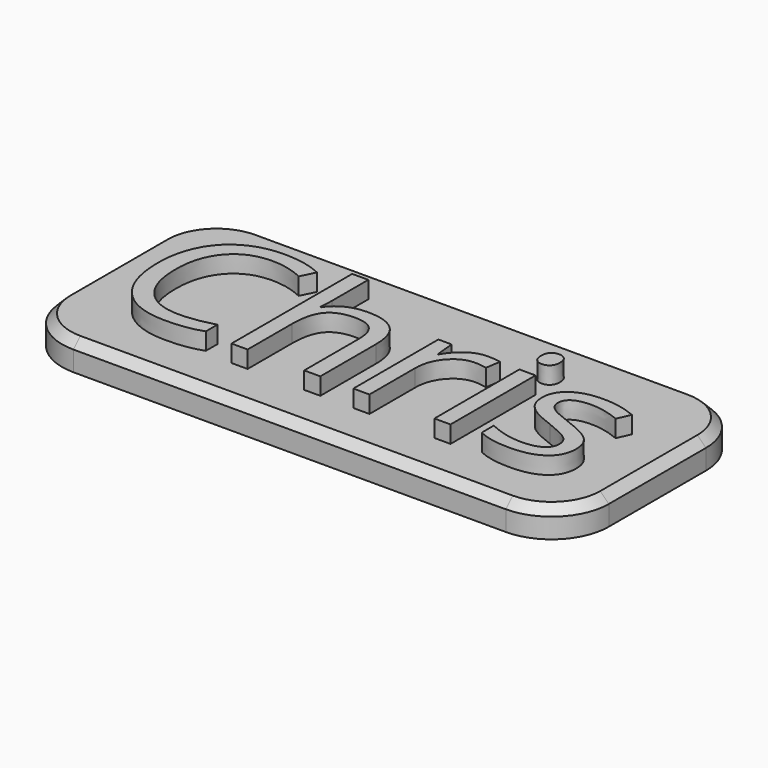
from build123d import *

# Parameters (mm, degrees)
F0_W         = 95.6249979794
F0_H         = 41.2499999501
F0_W_2       = 2.8157552083
F0_H_2       = 18.5818142361
F0_TEXT_SIZE = 34.7222222222
F1_DEPTH     = 5
F2_DEPTH     = 8
F3_R         = 10
F4_SIZE      = 1.5


# Not quite as in the source:
# - Text() gives the source's letters only with a copy of the font that has no kerning and outlines rounded to 1/6400 em; it was checked with that copy


with BuildPart() as f1:
    # F0 (on Top) → F1 (new body)
    with BuildSketch(Plane.XY):
        with Locations((6.9999974221, -3.5000005737)):
            Rectangle(F0_W, F0_H)
        with BuildLine():
            add(Edge.make_bspline(
                [(-14.9118961738, 5.2456596475), (-17.7276513822, 6.5640190225), (-20.5434065905, 6.5640190225)],
                knots=[0, 0, 0, 1, 1, 1], degree=2))
            add(Edge.make_bspline(
                [(-20.5434065905, 6.5640190225), (-24.6286930488, 6.5640190225), (-26.9941444377, 3.8432073905)],
                knots=[0, 0, 0, 1, 1, 1], degree=2))
            add(Edge.make_bspline(
                [(-26.9941444377, 3.8432073905), (-29.3595958266, 1.1223957586), (-29.3595958266, -3.6085070192)],
                knots=[0, 0, 0, 1, 1, 1], degree=2))
            add(Edge.make_bspline(
                [(-29.3595958266, -3.6085070192), (-29.3595958266, -8.4696181303), (-27.0782373197, -11.1253255956)],
                knots=[0, 0, 0, 1, 1, 1], degree=2))
            add(Edge.make_bspline(
                [(-27.0782373197, -11.1253255956), (-24.7968788127, -13.7810330609), (-20.5759586738, -13.7810330609)],
                knots=[0, 0, 0, 1, 1, 1], degree=2))
            add(Edge.make_bspline(
                [(-20.5759586738, -13.7810330609), (-17.9826427016, -13.7810330609), (-14.6569048544, -12.8478733387)],
                knots=[0, 0, 0, 1, 1, 1], degree=2))
            Line((-14.6569048544, -12.8478733387), (-14.6569048544, -15.370659797))
            add(Edge.make_bspline(
                [(-14.6569048544, -15.370659797), (-17.233944785, -16.3417969498), (-21.0154117988, -16.3417969498)],
                knots=[0, 0, 0, 1, 1, 1], degree=2))
            add(Edge.make_bspline(
                [(-21.0154117988, -16.3417969498), (-26.4895871461, -16.3417969498), (-29.4653900975, -13.0160591025)],
                knots=[0, 0, 0, 1, 1, 1], degree=2))
            add(Edge.make_bspline(
                [(-29.4653900975, -13.0160591025), (-32.4411930488, -9.6903212553), (-32.4411930488, -3.5705295887)],
                knots=[0, 0, 0, 1, 1, 1], degree=2))
            add(Edge.make_bspline(
                [(-32.4411930488, -3.5705295887), (-32.4411930488, 0.2597655502), (-31.0089013822, 3.1406249252)],
                knots=[0, 0, 0, 1, 1, 1], degree=2))
            add(Edge.make_bspline(
                [(-31.0089013822, 3.1406249252), (-29.5766097155, 6.0214843002), (-26.8720741252, 7.5812716266)],
                knots=[0, 0, 0, 1, 1, 1], degree=2))
            add(Edge.make_bspline(
                [(-26.8720741252, 7.5812716266), (-24.167538535, 9.141058953), (-20.50542916, 9.141058953)],
                knots=[0, 0, 0, 1, 1, 1], degree=2))
            add(Edge.make_bspline(
                [(-20.50542916, 9.141058953), (-16.6100298544, 9.141058953), (-13.6911930488, 7.7196179808)],
                knots=[0, 0, 0, 1, 1, 1], degree=2))
            Line((-13.6911930488, 7.7196179808), (-14.9118961738, 5.2456596475))
        make_face(mode=Mode.SUBTRACT)
        with BuildLine():
            add(Edge.make_bspline(
                [(16.9131906317, 1.9389105155), (18.3726090345, 2.9236110363), (20.11957084, 2.9236110363)],
                knots=[0, 0, 0, 1, 1, 1], degree=2))
            add(Edge.make_bspline(
                [(20.11957084, 2.9236110363), (21.3565500067, 2.9236110363), (22.3385378539, 2.7174478419)],
                knots=[0, 0, 0, 1, 1, 1], degree=2))
            Line((22.3385378539, 2.7174478419), (21.9479128539, 0.107855828))
            add(Edge.make_bspline(
                [(21.9479128539, 0.107855828), (20.7977392428, 0.3628471475), (19.9134076456, 0.3628471475)],
                knots=[0, 0, 0, 1, 1, 1], degree=2))
            add(Edge.make_bspline(
                [(19.9134076456, 0.3628471475), (17.6564632012, 0.3628471475), (16.0559857706, -1.46820754)],
                knots=[0, 0, 0, 1, 1, 1], degree=2))
            add(Edge.make_bspline(
                [(16.0559857706, -1.46820754), (14.45550834, -3.2992622275), (14.45550834, -6.0282118803)],
                knots=[0, 0, 0, 1, 1, 1], degree=2))
            Line((14.45550834, -6.0282118803), (14.45550834, -16.0000000748))
            Line((14.45550834, -16.0000000748), (11.6397531317, -16.0000000748))
            Line((11.6397531317, -16.0000000748), (11.6397531317, 2.5818141613))
            Line((11.6397531317, 2.5818141613), (13.9618017428, 2.5818141613))
            Line((13.9618017428, 2.5818141613), (14.2873225762, -0.8578559775))
            Line((14.2873225762, -0.8578559775), (14.4229562567, -0.8578559775))
            add(Edge.make_bspline(
                [(14.4229562567, -0.8578559775), (15.4537722289, 0.9542099947), (16.9131906317, 1.9389105155)],
                knots=[0, 0, 0, 1, 1, 1], degree=2))
        make_face(mode=Mode.SUBTRACT)
        with Locations((27.2240630275, -6.7090929567)):
            Rectangle(F0_W_2, F0_H_2, mode=Mode.SUBTRACT)
        with BuildLine():
            add(Edge.make_bspline(
                [(45.4233902845, -7.8619792414), (46.58441459, -9.0826823664), (46.58441459, -10.9327257692)],
                knots=[0, 0, 0, 1, 1, 1], degree=2))
            add(Edge.make_bspline(
                [(46.58441459, -10.9327257692), (46.58441459, -13.5260417414), (44.6529909789, -14.9339193456)],
                knots=[0, 0, 0, 1, 1, 1], degree=2))
            add(Edge.make_bspline(
                [(44.6529909789, -14.9339193456), (42.7215673678, -16.3417969498), (39.2276437567, -16.3417969498)],
                knots=[0, 0, 0, 1, 1, 1], degree=2))
            add(Edge.make_bspline(
                [(39.2276437567, -16.3417969498), (35.5329822984, -16.3417969498), (33.4659250067, -15.1699219498)],
                knots=[0, 0, 0, 1, 1, 1], degree=2))
            Line((33.4659250067, -15.1699219498), (33.4659250067, -12.5603299359))
            add(Edge.make_bspline(
                [(33.4659250067, -12.5603299359), (34.8059857706, -13.2384983387), (36.3386463609, -13.626410665)],
                knots=[0, 0, 0, 1, 1, 1], degree=2))
            add(Edge.make_bspline(
                [(36.3386463609, -13.626410665), (37.8713069512, -14.0143229914), (39.2981732706, -14.0143229914)],
                knots=[0, 0, 0, 1, 1, 1], degree=2))
            add(Edge.make_bspline(
                [(39.2981732706, -14.0143229914), (41.5008642428, -14.0143229914), (42.6863026109, -13.3117405262)],
                knots=[0, 0, 0, 1, 1, 1], degree=2))
            add(Edge.make_bspline(
                [(42.6863026109, -13.3117405262), (43.8717409789, -12.6091580609), (43.8717409789, -11.1660156998)],
                knots=[0, 0, 0, 1, 1, 1], degree=2))
            add(Edge.make_bspline(
                [(43.8717409789, -11.1660156998), (43.8717409789, -10.0809462553), (42.9331559095, -9.3105469498)],
                knots=[0, 0, 0, 1, 1, 1], degree=2))
            add(Edge.make_bspline(
                [(42.9331559095, -9.3105469498), (41.99457084, -8.5401476442), (39.26019584, -7.4876302831)],
                knots=[0, 0, 0, 1, 1, 1], degree=2))
            add(Edge.make_bspline(
                [(39.26019584, -7.4876302831), (36.6668798678, -6.5219184775), (35.5736724025, -5.800347297)],
                knots=[0, 0, 0, 1, 1, 1], degree=2))
            add(Edge.make_bspline(
                [(35.5736724025, -5.800347297), (34.4804649373, -5.0787761164), (33.9460682359, -4.1646051095)],
                knots=[0, 0, 0, 1, 1, 1], degree=2))
            add(Edge.make_bspline(
                [(33.9460682359, -4.1646051095), (33.4116715345, -3.2504341025), (33.4116715345, -1.9809028525)],
                knots=[0, 0, 0, 1, 1, 1], degree=2))
            add(Edge.make_bspline(
                [(33.4116715345, -1.9809028525), (33.4116715345, 0.2923176336), (35.2617149373, 1.607964335)],
                knots=[0, 0, 0, 1, 1, 1], degree=2))
            add(Edge.make_bspline(
                [(35.2617149373, 1.607964335), (37.11175834, 2.9236110363), (40.3289892428, 2.9236110363)],
                knots=[0, 0, 0, 1, 1, 1], degree=2))
            add(Edge.make_bspline(
                [(40.3289892428, 2.9236110363), (43.3292062567, 2.9236110363), (46.1992149373, 1.7029079113)],
                knots=[0, 0, 0, 1, 1, 1], degree=2))
            Line((46.1992149373, 1.7029079113), (45.1955257012, -0.5865886164))
            add(Edge.make_bspline(
                [(45.1955257012, -0.5865886164), (42.4014718817, 0.5635849947), (40.1282513956, 0.5635849947)],
                knots=[0, 0, 0, 1, 1, 1], degree=2))
            add(Edge.make_bspline(
                [(40.1282513956, 0.5635849947), (38.1262982706, 0.5635849947), (37.1090456664, -0.0630426095)],
                knots=[0, 0, 0, 1, 1, 1], degree=2))
            add(Edge.make_bspline(
                [(37.1090456664, -0.0630426095), (36.0917930623, -0.6896702137), (36.0917930623, -1.7910156998)],
                knots=[0, 0, 0, 1, 1, 1], degree=2))
            add(Edge.make_bspline(
                [(36.0917930623, -1.7910156998), (36.0917930623, -2.5397136164), (36.4742800414, -3.0632596234)],
                knots=[0, 0, 0, 1, 1, 1], degree=2))
            add(Edge.make_bspline(
                [(36.4742800414, -3.0632596234), (36.8567670206, -3.5868056303), (37.7031211873, -4.0615235123)],
                knots=[0, 0, 0, 1, 1, 1], degree=2))
            add(Edge.make_bspline(
                [(37.7031211873, -4.0615235123), (38.5494753539, -4.5362413942), (40.9583295206, -5.4368490331)],
                knots=[0, 0, 0, 1, 1, 1], degree=2))
            add(Edge.make_bspline(
                [(40.9583295206, -5.4368490331), (44.2623659789, -6.6412761164), (45.4233902845, -7.8619792414)],
                knots=[0, 0, 0, 1, 1, 1], degree=2))
        make_face(mode=Mode.SUBTRACT)
        with BuildLine():
            Line((5.86175834, -16.0000000748), (3.0460031317, -16.0000000748))
            Line((3.0460031317, -16.0000000748), (3.0460031317, -3.9774306303))
            add(Edge.make_bspline(
                [(3.0460031317, -3.9774306303), (3.0460031317, -1.7096354914), (2.0124744859, -0.58930129)],
                knots=[0, 0, 0, 1, 1, 1], degree=2))
            add(Edge.make_bspline(
                [(2.0124744859, -0.58930129), (0.97894584, 0.5310329113), (-1.2291704794, 0.5310329113)],
                knots=[0, 0, 0, 1, 1, 1], degree=2))
            add(Edge.make_bspline(
                [(-1.2291704794, 0.5310329113), (-4.1588579794, 0.5310329113), (-5.5070567641, -1.064019172)],
                knots=[0, 0, 0, 1, 1, 1], degree=2))
            add(Edge.make_bspline(
                [(-5.5070567641, -1.064019172), (-6.8552555488, -2.6590712553), (-6.8552555488, -6.2832031998)],
                knots=[0, 0, 0, 1, 1, 1], degree=2))
            Line((-6.8552555488, -6.2832031998), (-6.8552555488, -16.0000000748))
            Line((-6.8552555488, -16.0000000748), (-9.6710107572, -16.0000000748))
            Line((-9.6710107572, -16.0000000748), (-9.6710107572, 10.3834634669))
            Line((-9.6710107572, 10.3834634669), (-6.8552555488, 10.3834634669))
            Line((-6.8552555488, 10.3834634669), (-6.8552555488, 2.3973523558))
            add(Edge.make_bspline(
                [(-6.8552555488, 2.3973523558), (-6.8552555488, 0.9542099947), (-6.9908892294, 0.0047742308)],
                knots=[0, 0, 0, 1, 1, 1], degree=2))
            Line((-6.9908892294, 0.0047742308), (-6.8227034655, 0.0047742308))
            add(Edge.make_bspline(
                [(-6.8227034655, 0.0047742308), (-5.9926253405, 1.3448349947), (-4.4572520766, 2.1152343002)],
                knots=[0, 0, 0, 1, 1, 1], degree=2))
            add(Edge.make_bspline(
                [(-4.4572520766, 2.1152343002), (-2.9218788127, 2.8856336058), (-0.9579031183, 2.8856336058)],
                knots=[0, 0, 0, 1, 1, 1], degree=2))
            add(Edge.make_bspline(
                [(-0.9579031183, 2.8856336058), (2.4492149373, 2.8856336058), (4.1554866387, 1.26616746)],
                knots=[0, 0, 0, 1, 1, 1], degree=2))
            add(Edge.make_bspline(
                [(4.1554866387, 1.26616746), (5.86175834, -0.3532986859), (5.86175834, -3.8797743803)],
                knots=[0, 0, 0, 1, 1, 1], degree=2))
            Line((5.86175834, -3.8797743803), (5.86175834, -16.0000000748))
        make_face(mode=Mode.SUBTRACT)
        with BuildLine():
            add(Edge.make_bspline(
                [(26.0521880275, 6.2005207586), (25.5774701456, 6.6671006197), (25.5774701456, 7.6165363836)],
                knots=[0, 0, 0, 1, 1, 1], degree=2))
            add(Edge.make_bspline(
                [(25.5774701456, 7.6165363836), (25.5774701456, 8.5822481891), (26.0521880275, 9.0325520086)],
                knots=[0, 0, 0, 1, 1, 1], degree=2))
            add(Edge.make_bspline(
                [(26.0521880275, 9.0325520086), (26.5269059095, 9.482855828), (27.2430517428, 9.482855828)],
                knots=[0, 0, 0, 1, 1, 1], degree=2))
            add(Edge.make_bspline(
                [(27.2430517428, 9.482855828), (27.9212201456, 9.482855828), (28.4122140692, 9.0244139877)],
                knots=[0, 0, 0, 1, 1, 1], degree=2))
            add(Edge.make_bspline(
                [(28.4122140692, 9.0244139877), (28.9032079928, 8.5659721475), (28.9032079928, 7.6165363836)],
                knots=[0, 0, 0, 1, 1, 1], degree=2))
            add(Edge.make_bspline(
                [(28.9032079928, 7.6165363836), (28.9032079928, 6.6671006197), (28.4122140692, 6.2005207586)],
                knots=[0, 0, 0, 1, 1, 1], degree=2))
            add(Edge.make_bspline(
                [(28.4122140692, 6.2005207586), (27.9212201456, 5.7339408975), (27.2430517428, 5.7339408975)],
                knots=[0, 0, 0, 1, 1, 1], degree=2))
            add(Edge.make_bspline(
                [(27.2430517428, 5.7339408975), (26.5269059095, 5.7339408975), (26.0521880275, 6.2005207586)],
                knots=[0, 0, 0, 1, 1, 1], degree=2))
        make_face(mode=Mode.SUBTRACT)
        with Locations((-34.5625038127, -16.0000000748)):
            Text('Chris', F0_TEXT_SIZE, font='Open Sans', text_align=(TextAlign.LEFT, TextAlign.BOTTOM))
    extrude(amount=F1_DEPTH)

    # F0 (on Top) → F2 (join)
    with BuildSketch(Plane.XY):
        with Locations((-34.5625038127, -16.0000000748)):
            Text('Chris', F0_TEXT_SIZE, font='Open Sans', text_align=(TextAlign.LEFT, TextAlign.BOTTOM))
    extrude(amount=F2_DEPTH)

    # F3
    f3_edges = [f1.edges().sort_by_distance(p)[0] for p in [
        (-40.812502, -24.125001, 2.5),
        (54.812496, -24.125001, 2.5),
        (54.812496, 17.124999, 2.5),
        (-40.812502, 17.124999, 2.5),
    ]]
    fillet(f3_edges, radius=F3_R)

    # F4
    f4_edges = [f1.edges().sort_by_distance(p)[0] for p in [
        (6.999997, -24.125001, 5),
    ]]
    chamfer(f4_edges, length=F4_SIZE)


solid = f1.part
